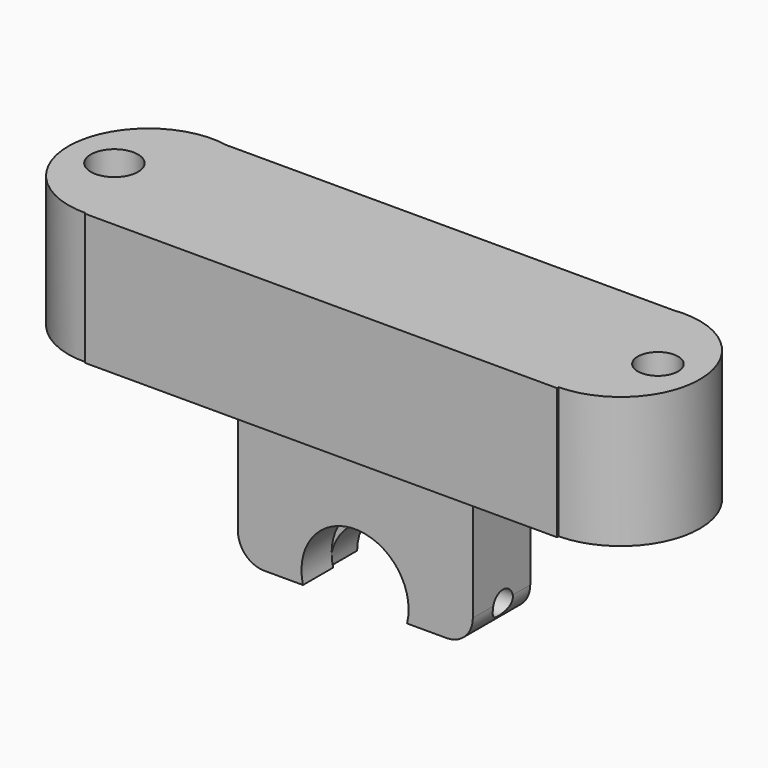
from build123d import *

# Parameters (mm, degrees)
F1_R         = 15.4658150948
F3_DEPTH     = 25.4
F0_W         = 91.367084533
F0_H         = 30.8810528368
F4_DEPTH     = 25.4
F2_R         = 15.313452945
F5_DEPTH     = 25.4
F6_R         = 3.9725855112
F7_DEPTH     = 25.4
F8_R         = 4.5697295071
F9_DEPTH     = 26.67
F10_R        = 3.9038322972
F11_DEPTH    = 30.988
F12_W        = 45.4270541668
F12_H        = 13.8839902356
F13_DEPTH    = 29.718
F15_R        = 10.7036365959
F16_DEPTH    = 25.4
F17_R        = 10.3585042146
F18_DEPTH    = 46.736
F14_R        = 2.4093664871
F19_DEPTH    = 44.196
F20_R        = 5.08
F21_T1_DEPTH = 39.2839902356


# Not quite as in the source:
# - a fillet or chamfer that OpenCascade refuses, or shapes differently, is made with other operations: its cross-section is extruded or revolved along the edge and cut away or added


with BuildPart() as f3:
    # F1 (on Top) → F3 (new body)
    with BuildSketch(Plane.XY):
        with Locations((-45.811150223, 0)):
            Circle(F1_R)
    extrude(amount=F3_DEPTH)

    # F0 (on Top) → F4 (join)
    with BuildSketch(Plane.XY):
        with Locations((0.1276079565, -0.2552149817)):
            Rectangle(F0_W, F0_H)
    extrude(amount=F4_DEPTH)

    # F2 (on Top) → F5 (join)
    with BuildSketch(Plane.XY):
        with Locations((45.55593431, 0)):
            Circle(F2_R)
    extrude(amount=F5_DEPTH)

    # F6 (on Top) → F7 (cut)
    with BuildSketch(Plane.XY):
        with Locations((-53.0294403434, 0)):
            Circle(F6_R)
    extrude(amount=-F7_DEPTH, mode=Mode.SUBTRACT)

    # F8 (on Top) → F9 (cut)
    with BuildSketch(Plane.XY):
        with Locations((-52.3779653013, 0)):
            Circle(F8_R)
    extrude(amount=F9_DEPTH, mode=Mode.SUBTRACT)

    # F10 (on Top) → F11 (cut)
    with BuildSketch(Plane.XY):
        with Locations((52.7567230165, 0)):
            Circle(F10_R)
    extrude(amount=F11_DEPTH, mode=Mode.SUBTRACT)

    # F12 (on Top) → F13 (join)
    with BuildSketch(Plane.XY):
        with Locations((0.0732727349, -0.3520357423)):
            Rectangle(F12_W, F12_H)
    extrude(amount=-F13_DEPTH)

    # F15 (on Front) → F16 (cut)
    with BuildSketch(Plane.XZ):
        with Locations((0, -29.8675838858)):
            Circle(F15_R)
    extrude(amount=-F16_DEPTH, mode=Mode.SUBTRACT)

    # F17 (on Front) → F18 (cut)
    with BuildSketch(Plane.XZ):
        with Locations((0, -27.270803228)):
            Circle(F17_R)
    extrude(amount=F18_DEPTH, mode=Mode.SUBTRACT)

    # F14 (on Right) → F19 (cut)
    with BuildSketch(Plane.YZ):
        with Locations((0, -25.1646973193)):
            Circle(F14_R)
    extrude(amount=F19_DEPTH, mode=Mode.SUBTRACT)

    # F20
    f20_edges = [f3.edges().sort_by_distance(p)[0] for p in [
        (-22.640254, -0.352036, -29.718),
    ]]
    fillet(f20_edges, radius=F20_R)

    # F21: fillet of radius 5.08 on 1 edges, made by hand

    # F21_s2 → F21_t1 (cut)
    with BuildSketch(Plane.XZ.offset(-19.2899593756)):
        with BuildLine():
            ThreePointArc((22.7867998183, -24.638), (21.2989022667, -28.2301024484), (17.7067998183, -29.718))
            Line((17.7067998183, -29.718), (22.7867998183, -29.718))
            Line((22.7867998183, -29.718), (22.7867998183, -24.638))
        make_face()
    extrude(amount=F21_T1_DEPTH, mode=Mode.SUBTRACT)


solid = f3.part
